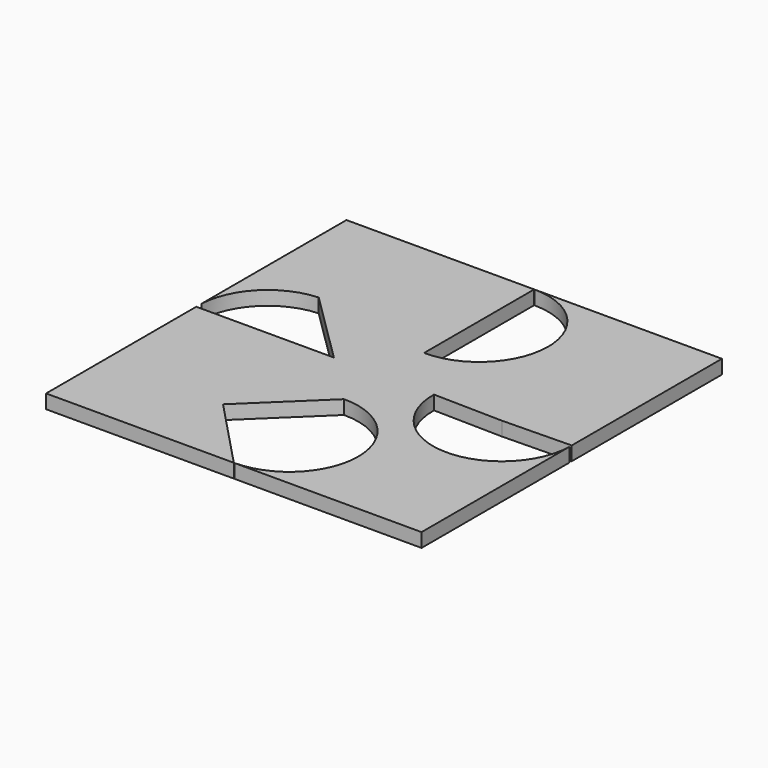
from build123d import *

# Parameters (mm, degrees)
F1_DEPTH = 6.604


with BuildPart() as f1:
    # F0 (on Top) → F1 (new body)
    with BuildSketch(Plane.XY):
        Polygon((-88.9, 88.9), (0, 0), (88.9, 88.9), (0, 88.9), align=None)
        with BuildLine():
            ThreePointArc((0, 23.6728), (-32.5308292905, 56.2864), (0, 88.9))
            ThreePointArc((0, 88.9), (22.0701917215, 80.3739843781), (32.5687625572, 59.1710054502))
            ThreePointArc((32.5687625572, 59.1710054502), (32.6646109516, 57.7301179639), (32.6965813095, 56.2864))
            ThreePointArc((32.6965813095, 56.2864), (23.1149284543, 33.1957453196), (0, 23.6728))
        make_face(mode=Mode.SUBTRACT)
        with BuildLine():
            Line((88.9, 88.9), (0, 0))
            Line((0, 0), (88.9, -88.9))
            Line((88.9, -88.9), (88.9, -1.303055018))
            ThreePointArc((88.9, -1.303055018), (78.2779390849, -24.7410549975), (53.9692081511, -33.1822410226))
            ThreePointArc((53.9692081511, -33.1822410226), (32.2033809996, -22.6365581058), (23.6858169762, 0))
            ThreePointArc((23.6858169762, 0), (56.2929084881, 31.962072491), (88.9, 0))
            Line((88.9, 0), (88.9, 88.9))
        make_face()
        with BuildLine():
            Line((-88.9, -88.9), (0, -88.9))
            ThreePointArc((0, -88.9), (-23.4333822085, -78.7489741197), (-32.3691311793, -54.8257820567))
            ThreePointArc((-32.3691311793, -54.8257820567), (-22.4036802199, -32.787394799), (0, -23.6728))
            ThreePointArc((0, -23.6728), (23.1989938683, -33.1496268937), (32.826729568, -56.2864))
            ThreePointArc((32.826729568, -56.2864), (23.3492107959, -79.2729561788), (0.4248753792, -88.9))
            Line((0.4248753792, -88.9), (88.9, -88.9))
            Line((88.9, -88.9), (0, 0))
            Line((0, 0), (-88.9, -88.9))
        make_face()
        with BuildLine():
            Line((-88.9, 0), (-88.9, -88.9))
            Line((-88.9, -88.9), (0, 0))
            Line((0, 0), (-88.9, 88.9))
            Line((-88.9, 88.9), (-88.9, 3.0109182433))
            ThreePointArc((-88.9, 3.0109182433), (-79.5055607914, 24.4438044642), (-58.1749416888, 34.0681895614))
            ThreePointArc((-58.1749416888, 34.0681895614), (-33.9222205657, 25.2151766333), (-23.7036289165, 1.5054591217))
            ThreePointArc((-23.7036289165, 1.5054591217), (-23.7123207699, 0.7525289094), (-23.7383916974, 0))
            ThreePointArc((-23.7383916974, 0), (-56.3191958487, -31.1101078106), (-88.9, 0))
        make_face()
        with BuildLine():
            Line((0, 23.6728), (0, 88.9))
            ThreePointArc((0, 88.9), (-32.5308292905, 56.2864), (0, 23.6728))
        make_face()
        with BuildLine():
            Line((56.2929084881, -0.651527509), (88.9, 0))
            ThreePointArc((88.9, 0), (56.2929084881, 31.962072491), (23.6858169762, 0))
            Line((23.6858169762, 0), (56.2929084881, -0.651527509))
        make_face()
        with BuildLine():
            Line((-23.7383916974, 0), (-88.9, 0))
            ThreePointArc((-88.9, 0), (-56.3191958487, -31.1101078106), (-23.7383916974, 0))
        make_face()
        with BuildLine():
            Line((-58.1749416888, 34.0681895614), (-23.7383916974, 0))
            ThreePointArc((-23.7383916974, 0), (-23.7123207699, 0.7525289094), (-23.7036289165, 1.5054591217))
            ThreePointArc((-23.7036289165, 1.5054591217), (-33.9222205657, 25.2151766333), (-58.1749416888, 34.0681895614))
        make_face()
        with BuildLine():
            ThreePointArc((-32.3691311793, -54.8257820567), (-23.4333822085, -78.7489741197), (0, -88.9))
            Line((0, -88.9), (-32.3691311793, -54.8257820567))
        make_face()
        with BuildLine():
            ThreePointArc((0, -23.6728), (-22.4036802199, -32.787394799), (-32.3691311793, -54.8257820567))
            Line((-32.3691311793, -54.8257820567), (0, -23.6728))
        make_face()
    extrude(amount=-F1_DEPTH)


solid = f1.part
